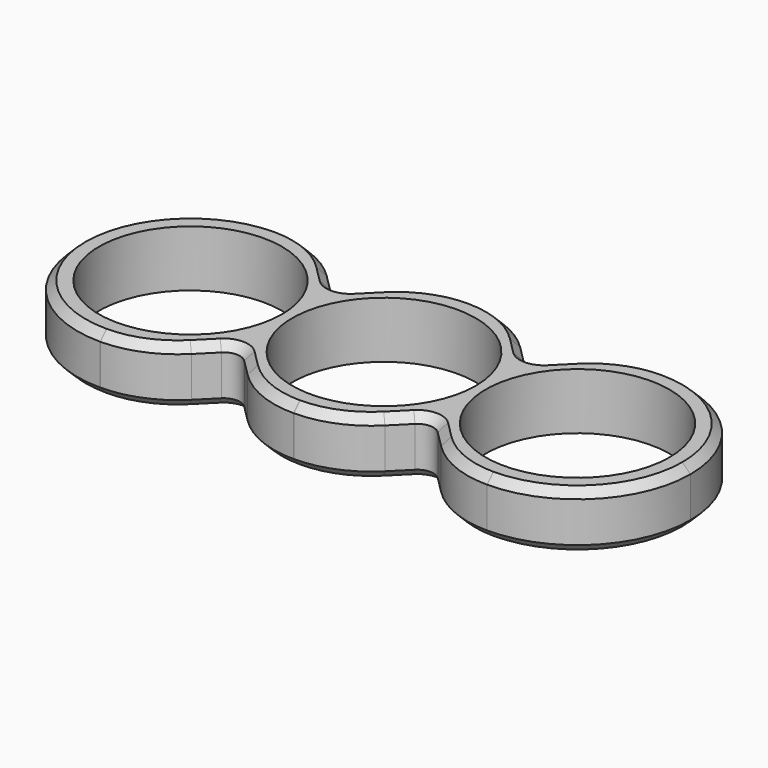
from build123d import *

# Parameters (mm, degrees)
F0_W     = 76
F0_H     = 28
F0_R     = 11.35
F0_R_2   = 11.375
F0_R_3   = 11.4
F1_DEPTH = 7
F3_DEPTH = 7.001
F4_R     = 13.99999
F5_R     = 12
F6_R     = 2
F7_SIZE  = 1


# Not quite as in the source:
# - a fillet or chamfer is up to 0.001 mm smaller than in the source, because OpenCascade refuses the exact size


with BuildPart() as f1:
    # F0 (on Top) → F1 (new body)
    with BuildSketch(Plane.XY):
        Rectangle(F0_W, F0_H)
        with Locations((-24, 0)):
            Circle(F0_R, mode=Mode.SUBTRACT)
        Circle(F0_R_2, mode=Mode.SUBTRACT)
        with Locations((24, 0)):
            Circle(F0_R_3, mode=Mode.SUBTRACT)
    extrude(amount=F1_DEPTH)

    # F2 (on face) → F3 (cut, through all)
    with BuildSketch(Plane.XY.offset(7)):
        Polygon((-5.0125, 14), (-19.0125, 14), (-12.0125, 7), align=None)
        Polygon((18.9875, 14), (4.9875, 14), (11.9875, 7), align=None)
        Polygon((11.9875, -7), (4.9875, -14), (18.9875, -14), align=None)
        Polygon((-5.0125, -14), (-12.0125, -7), (-19.0125, -14), align=None)
    extrude(amount=-F3_DEPTH, mode=Mode.SUBTRACT)

    # F4 (radius 14 in the source; OpenCascade refuses exactly that, so slightly less here)
    f4_edges = [f1.edges().sort_by_distance(p)[0] for p in [
        (-38, -14, 3.5),
        (-38, 14, 3.5),
        (38, -14, 3.5),
        (38, 14, 3.5),
    ]]
    fillet(f4_edges, radius=F4_R)

    # F5
    f5_edges = [f1.edges().sort_by_distance(p)[0] for p in [
        (-19.0125, -14, 3.5),
        (-5.0125, -14, 3.5),
        (4.9875, -14, 3.5),
        (18.9875, -14, 3.5),
        (18.9875, 14, 3.5),
        (4.9875, 14, 3.5),
        (-5.0125, 14, 3.5),
        (-19.0125, 14, 3.5),
    ]]
    fillet(f5_edges, radius=F5_R)

    # F6
    f6_edges = [f1.edges().sort_by_distance(p)[0] for p in [
        (-12.0125, -7, 3.5),
        (11.9875, -7, 3.5),
        (-12.0125, 7, 3.5),
        (11.9875, 7, 3.5),
    ]]
    fillet(f6_edges, radius=F6_R)

    # F7
    f7_edges = [f1.edges().sort_by_distance(p)[0] for p in [
        (-4.634138, -13.086554, 7),
        (-4.634138, -13.086554, 0),
    ]]
    chamfer(f7_edges, length=F7_SIZE)


solid = f1.part
